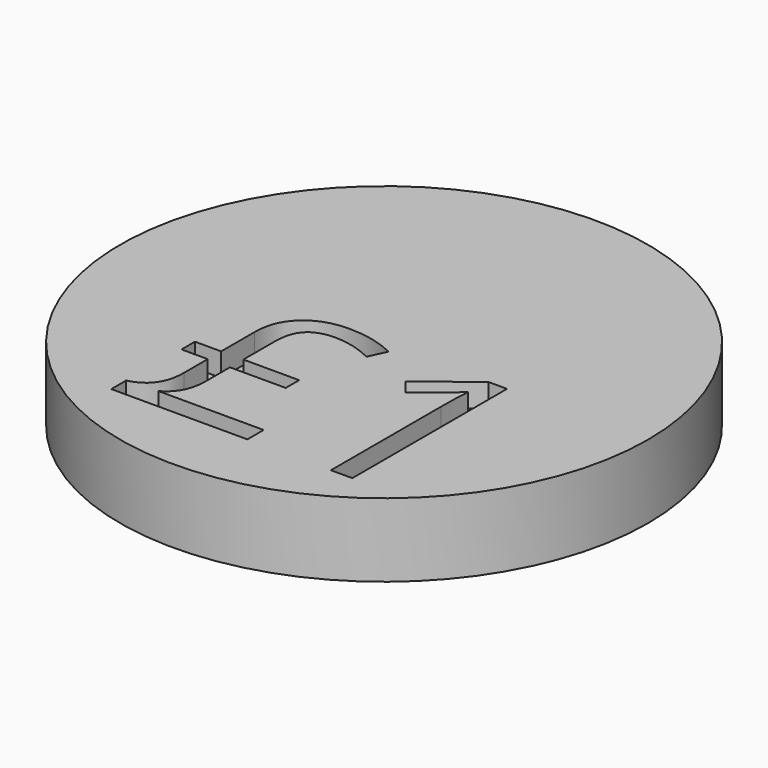
from build123d import *

# Parameters (mm, degrees)
F0_R         = 11.27
F1_DEPTH     = 3.14
F2_TEXT_SIZE = 11.5640744615
F3_DEPTH     = 1


# Not quite as in the source:
# - Text() gives the source's letters only with a copy of the font that has no kerning and outlines rounded to 1/6400 em; it was checked with that copy


with BuildPart() as f1:
    # F0 (on Top) → F1 (new body)
    with BuildSketch(Plane.XY):
        Circle(F0_R)
    extrude(amount=F1_DEPTH)

    # F2 (on face) → F3 (cut)
    with BuildSketch(Plane.XY.offset(3.14)):
        with Locations((-5.3427238017, -8.3261336123)):
            Text('£1', F2_TEXT_SIZE, font='Open Sans', text_align=(TextAlign.LEFT, TextAlign.BOTTOM))
    extrude(amount=-F3_DEPTH, mode=Mode.SUBTRACT)


solid = f1.part
